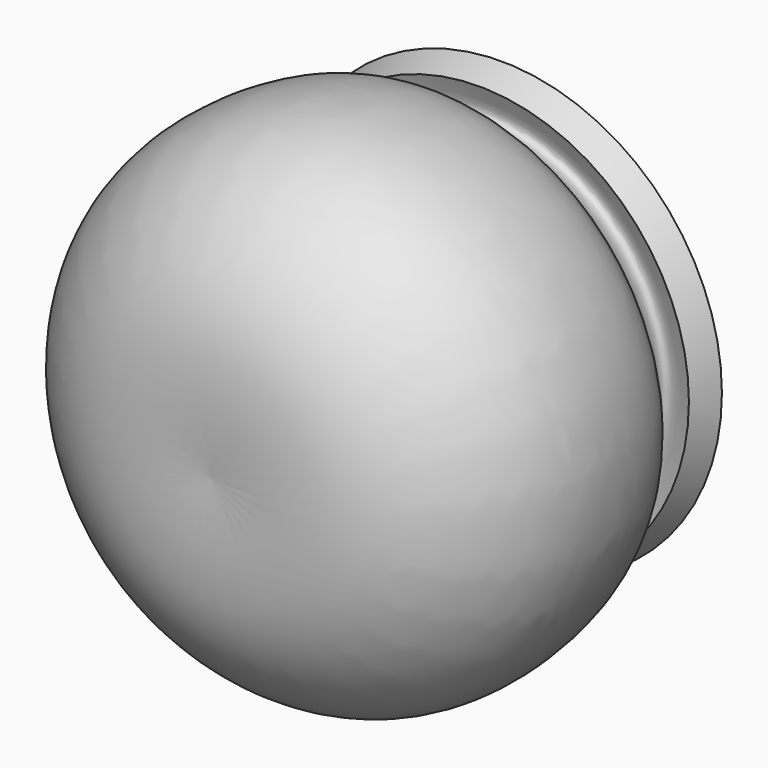
from build123d import *


# Not quite as in the source:
# - the dataset's text gives a spline's control points without its knots; the knots are read off the source's solid


with BuildPart() as f1:
    # F0 (on Top) → F1 (revolve)
    with BuildSketch(Plane.XY):
        with BuildLine():
            add(Edge.make_bspline(
                [(0.433260443, -40.4515990364), (0.2888402953, -40.4056839782), (0.1444201477, -40.3597689199), (0, -40.3138538617)],
                knots=[0, 0, 0, 0, 0.4546298985, 0.4546298985, 0.4546298985, 0.4546298985], degree=3))
            Line((0, -40.3138538617), (0, -46.7868000269))
            add(Edge.make_bspline(
                [(0, -46.7868000269), (10.5945035996, -47.5113515178), (31.2614693132, -48.9247524082), (53.8313986883, -27.403185884), (55.4492993068, -4.5930863041), (50.5842542409, 14.2871507074), (39.1286823085, 19.8718812054), (37.38112024, 27.7693327876), (42.2150864799, 25.8628705939), (44.8056012392, 24.8412005603)],
                knots=[0, 0, 0, 0, 0.1981094962, 0.386457197, 0.555324633, 0.7086984959, 0.8332501339, 0.9106390141, 1, 1, 1, 1], degree=3))
            add(Edge.make_bspline(
                [(47.1353294975, 30.7483870686), (46.3587534114, 28.7793248992), (45.5821773253, 26.8102627297), (44.8056012392, 24.8412005603)],
                knots=[0, 0, 0, 0, 6.3499989134, 6.3499989134, 6.3499989134, 6.3499989134], degree=3))
            add(Edge.make_bspline(
                [(0.433260443, -40.4515990364), (3.7756366932, -40.6801820628), (8.666360415, -41.0116022642), (14.7944751142, -41.0567897268), (19.1516833363, -40.8140917306), (22.5529195453, -40.3252739828), (25.1268247412, -39.7347796772), (26.6751699787, -39.2770773408), (27.8788481623, -38.8541729721), (29.0610668553, -38.3914555007), (30.5315379186, -37.72550391), (32.2652758131, -36.7970269219), (34.5224179127, -35.3974997585), (37.2100649682, -33.3704114924), (40.1275552475, -30.5846742395), (42.6483764666, -27.5518860062), (44.6963452649, -24.3843515033), (46.1944660925, -21.2275902028), (47.2443303131, -17.9725223075), (47.8981523378, -14.6085979841), (48.1471925287, -11.7088350573), (48.1878187097, -9.3384878313), (48.1440828343, -7.5378912221), (48.0314274413, -5.719796377), (47.8558090166, -3.8803434626), (47.6242865651, -2.0805766672), (47.2368333393, 0.2471480689), (46.7290003703, 2.4320459679), (46.1055054217, 4.4057394912), (45.5848011329, 5.7636851265), (45.0177831316, 6.9840609756), (44.514723707, 7.8760034003), (44.0997159501, 8.5110194841), (43.8363913959, 8.8750130457), (43.6239053337, 9.1467780827), (43.4108221535, 9.4052499666), (43.1182242195, 9.7342740767), (42.7277998914, 10.1355146548), (42.1535371759, 10.682234703), (41.3379187834, 11.3891028711), (40.2195123166, 12.2870977042), (38.9846108112, 13.2590911182), (37.6579278234, 14.3475618591), (36.4994143181, 15.4071333408), (35.5656875473, 16.3939564688), (34.9887784283, 17.0800245117), (34.5382992666, 17.6774733356), (34.1008141361, 18.3068501511), (33.6129423218, 19.1041954028), (33.1071657267, 20.0903580517), (32.6807117161, 21.1100324728), (32.334960527, 22.1789010297), (32.0800549683, 23.3239343668), (31.943262175, 24.5904063688), (31.9806357318, 25.8060201281), (32.1777594121, 26.9125009309), (32.4422971836, 27.8118177568), (32.8621961764, 28.769950605), (33.3752429791, 29.5885679795), (33.8935529597, 30.2222546466), (34.3354584526, 30.6770343379), (34.8237788995, 31.0972503356), (35.4968038996, 31.5807475524), (36.3564407324, 32.0451505597), (37.3370625298, 32.3999145902), (38.2299308415, 32.6018130811), (39.2936808847, 32.7276403264), (40.4068296968, 32.7094008179), (41.510869344, 32.5660506713), (42.474448897, 32.3612391461), (43.3522049229, 32.121582243), (44.1755154179, 31.8599528589), (44.9611129461, 31.5847503051), (45.9683593413, 31.2089528336), (46.6823712776, 30.927028722), (47.1353294975, 30.7483870686)],
                knots=[0, 0, 0, 0, 0.0625, 0.09375, 0.125, 0.15625, 0.171875, 0.1875, 0.1953125, 0.203125, 0.21875, 0.234375, 0.25, 0.28125, 0.3125, 0.34375, 0.375, 0.40625, 0.4375, 0.46875, 0.5, 0.515625, 0.53125, 0.546875, 0.5625, 0.578125, 0.59375, 0.625, 0.640625, 0.65625, 0.671875, 0.6875, 0.6953125, 0.703125, 0.70703125, 0.7109375, 0.71875, 0.7265625, 0.734375, 0.75, 0.765625, 0.78125, 0.796875, 0.8125, 0.8203125, 0.828125, 0.83203125, 0.8359375, 0.84375, 0.8515625, 0.859375, 0.8671875, 0.875, 0.8828125, 0.890625, 0.89453125, 0.8984375, 0.90234375, 0.90625, 0.908203125, 0.91015625, 0.912109375, 0.9140625, 0.91796875, 0.921875, 0.92578125, 0.9296875, 0.9375, 0.9453125, 0.953125, 0.9609375, 0.96875, 0.9765625, 0.984375, 1, 1, 1, 1], degree=3))
        make_face()
    revolve(axis=Axis((0, -0.7619988173, 0), (0, -1, 0)))


solid = f1.part
